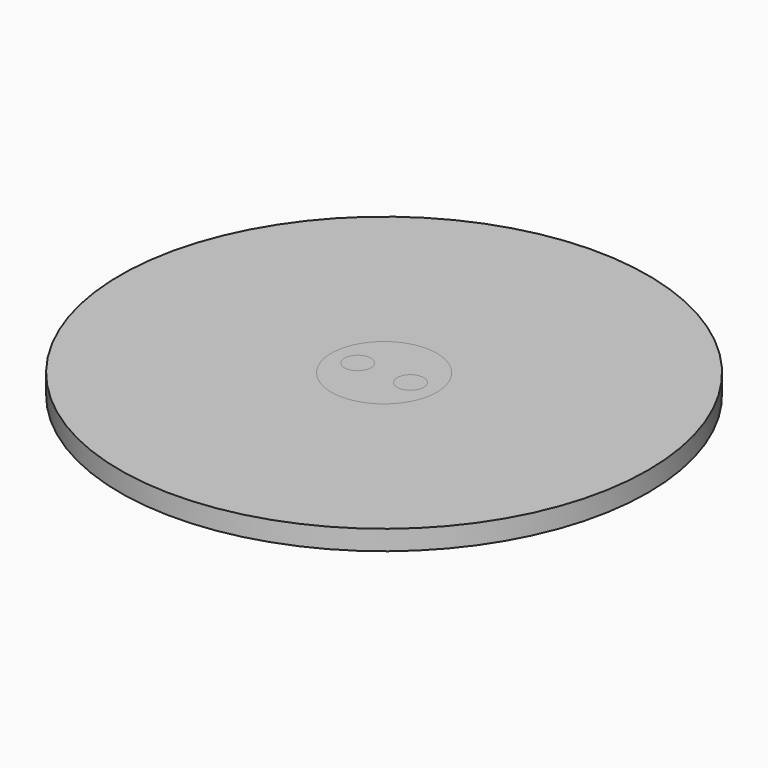
from build123d import *

# Parameters (mm, degrees)
F0_R      = 20
F1_DEPTH  = 1.5
F2_R      = 5.5
F3_DEPTH  = 5
F4_R      = 4
F5_DEPTH  = 25
F6_R      = 4
F7_DEPTH  = 5
F8_R      = 1
F9_DEPTH  = 8
F11_DEPTH = 3
F12_DEPTH = 25
F13_W     = 2
F13_H     = 0.5
F14_DEPTH = 12.5


with BuildPart() as f1:
    # F0 (on Top) → F1 (new body)
    with BuildSketch(Plane.XY):
        Circle(F0_R)
    extrude(amount=F1_DEPTH)

    # F2 (on face) → F3 (join)
    with BuildSketch(Plane.XY.offset(1.5)):
        Circle(F2_R)
    extrude(amount=-F3_DEPTH)

    # F4 (on face) → F5 (cut)
    with BuildSketch(Plane.XY.offset(1.5)):
        Circle(F4_R)
    extrude(amount=-F5_DEPTH, mode=Mode.SUBTRACT)


with BuildPart() as f7:
    # F6 (on face) → F7 (new body)
    with BuildSketch(Plane.XY.offset(1.5)):
        Circle(F6_R)
    extrude(amount=-F7_DEPTH)

    # F8 (on face) → F12 (cut)
    with BuildSketch(Plane.XY.offset(1.5)):
        with Locations((-2, 0)):
            Circle(F8_R)
        with Locations((2, 0)):
            Circle(F8_R)
    extrude(amount=-F12_DEPTH, mode=Mode.SUBTRACT)


with BuildPart() as f9:
    # F8 (on face) → F9 (new body)
    with BuildSketch(Plane.XY.offset(1.5)):
        with Locations((-2, 0)):
            Circle(F8_R)
    extrude(amount=-F9_DEPTH)


with BuildPart() as f9b:
    # F8 (on face) → F9, piece 2 (new body)
    with BuildSketch(Plane.XY.offset(1.5)):
        with Locations((2, 0)):
            Circle(F8_R)
    extrude(amount=-F9_DEPTH)


with BuildPart() as f11_tool:
    # F10 (on face) → F11 (new body)
    with BuildSketch(Plane(origin=(0, 0, -6.5), x_dir=(1, 0, 0), z_dir=(0, 0, -1))):
        with BuildLine():
            Line((2.6708203932, 0.2), (2.9797958971, 0.2))
            ThreePointArc((2.9797958971, 0.2), (2, 1), (1.0202041029, 0.2))
            Line((1.0202041029, 0.2), (1.3291796068, 0.2))
            ThreePointArc((1.3291796068, 0.2), (2, -0.7), (2.6708203932, 0.2))
        make_face()
        with BuildLine():
            Line((-2.9797958971, 0.2), (-2.6708203932, 0.2))
            ThreePointArc((-2.6708203932, 0.2), (-2, -0.7), (-1.3291796068, 0.2))
            Line((-1.3291796068, 0.2), (-1.0202041029, 0.2))
            ThreePointArc((-1.0202041029, 0.2), (-2, 1), (-2.9797958971, 0.2))
        make_face()
    extrude(amount=-F11_DEPTH)


with BuildPart() as f9_1:
    add(f9.part)

    # F11: cut by f11_tool
    add(f11_tool.part, mode=Mode.SUBTRACT)


with BuildPart() as f9b_1:
    add(f9b.part)

    # F11: cut by f11_tool
    add(f11_tool.part, mode=Mode.SUBTRACT)


with BuildPart() as f14_tool:
    # F13 (on Right) → F14 (new body, symmetric)
    with BuildSketch(Plane.YZ):
        with Locations((-0.6, -3.75)):
            Rectangle(F13_W, F13_H)
    extrude(amount=F14_DEPTH, both=True)


with BuildPart() as f9_2:
    add(f9_1.part)

    # F14: cut by f14_tool
    add(f14_tool.part, mode=Mode.SUBTRACT)


with BuildPart() as f9b_2:
    add(f9b_1.part)

    # F14: cut by f14_tool
    add(f14_tool.part, mode=Mode.SUBTRACT)


solid = Compound([f1.part, f7.part, f9_2.part, f9b_2.part])
